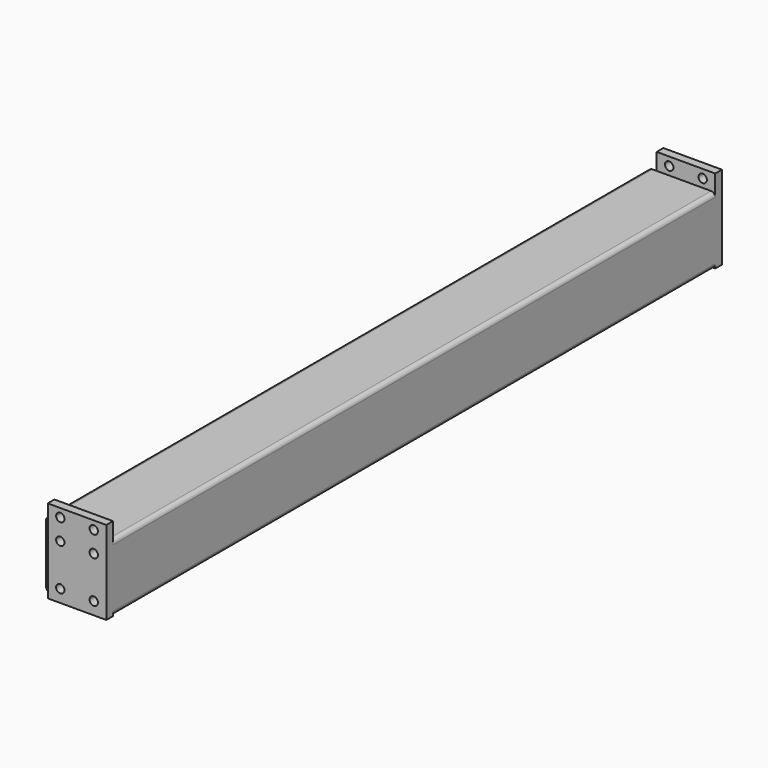
from build123d import *

# Parameters (mm, degrees)
F0_W     = 74
F0_H     = 74
F1_DEPTH = 900
F2_W     = 67
F2_H     = 74
F3_DEPTH = 10
F4_R     = 5
F5_DEPTH = 25


# Not quite as in the source:
# - a pattern or mirror of a feature is missing from the dataset's text; its kind, count and spacing are read off the source's solid


with BuildPart() as f1:
    # F0 (on Front) → F1 (new body)
    with BuildSketch(Plane.XZ):
        with BuildLine():
            ThreePointArc((40, 35), (38.5355339059, 38.5355339059), (35, 40))
            Line((35, 40), (-35, 40))
            ThreePointArc((-35, 40), (-38.5355339059, 38.5355339059), (-40, 35))
            Line((-40, 35), (-40, -35))
            ThreePointArc((-40, -35), (-38.5355339059, -38.5355339059), (-35, -40))
            Line((-35, -40), (35, -40))
            ThreePointArc((35, -40), (38.5355339059, -38.5355339059), (40, -35))
            Line((40, -35), (40, 35))
        make_face()
        Rectangle(F0_W, F0_H, mode=Mode.SUBTRACT)
    extrude(amount=F1_DEPTH)

    # F2 (on face) → F3 (join)
    with BuildSketch(Plane.XZ.offset(900)):
        with Locations((3.5, 0)):
            Rectangle(F2_W, F2_H)
        with BuildLine():
            Line((-30, -37), (-30, -40))
            Line((-30, -40), (35, -40))
            ThreePointArc((35, -40), (38.5355339059, -38.5355339059), (40, -35))
            Line((40, -35), (40, 35))
            ThreePointArc((40, 35), (38.5355339059, 38.5355339059), (35, 40))
            Line((35, 40), (-30, 40))
            Line((-30, 40), (-30, 37))
            Line((-30, 37), (37, 37))
            Line((37, 37), (37, -37))
            Line((37, -37), (-30, -37))
        make_face()
        with BuildLine():
            ThreePointArc((40, -35), (38.5355339059, -38.5355339059), (35, -40))
            Line((35, -40), (40, -40))
            Line((40, -40), (40, -35))
        make_face()
        with BuildLine():
            ThreePointArc((35, 40), (38.5355339059, 38.5355339059), (40, 35))
            Line((40, 35), (40, 60))
            Line((40, 60), (-30, 60))
            Line((-30, 60), (-30, 40))
            Line((-30, 40), (35, 40))
        make_face()
    f3 = extrude(amount=F3_DEPTH)

    # F3_copies: F3 across plane
    add(f3.mirror(Plane.ZX.offset(-450)))

    # F4 (on face) → F5 (cut)
    with BuildSketch(Plane(origin=(0, -900, 0), x_dir=(-1, 0, 0), z_dir=(0, 1, 0))):
        with Locations((-25, 50)):
            Circle(F4_R)
        with Locations((15, 50)):
            Circle(F4_R)
        with Locations((15, 25)):
            Circle(F4_R)
        with Locations((-25, 25)):
            Circle(F4_R)
        with Locations((-25, -25)):
            Circle(F4_R)
        with Locations((15, -25)):
            Circle(F4_R)
    f5 = extrude(amount=-F5_DEPTH, mode=Mode.SUBTRACT)

    # F5_copies: F5 across plane
    add(f5.mirror(Plane.ZX.offset(-450)), mode=Mode.SUBTRACT)


solid = f1.part
